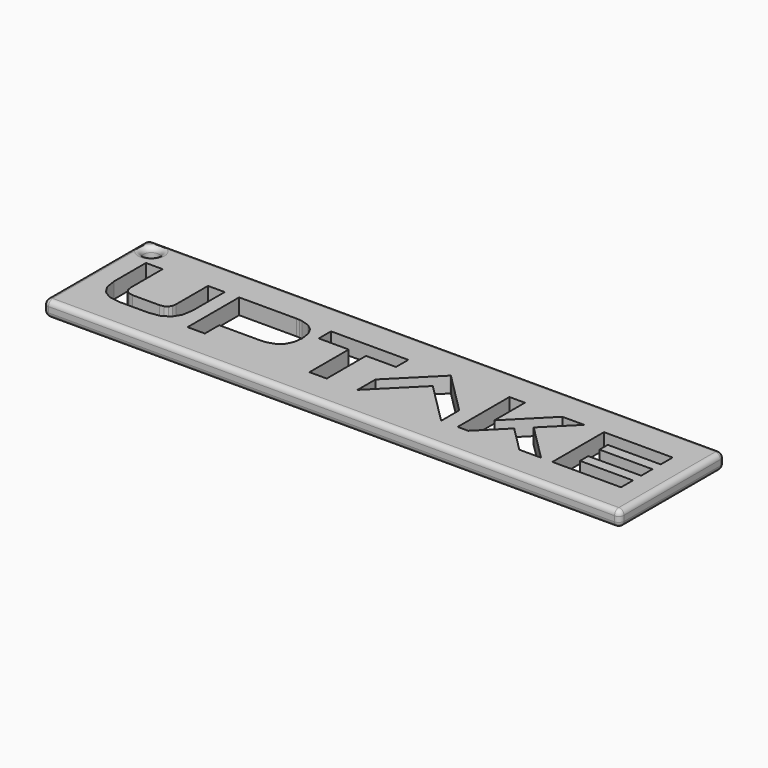
from build123d import *

# Parameters (mm, degrees)
F0_W         = 139.7
F0_H         = 31.75
F1_DEPTH     = 3.81
F3_D         = 3.81
F4_T1_DEPTH  = 137.1580686292
F4_T3_DEPTH  = 29.2080686292
F4_T5_DEPTH  = 1.2680686292
F4_S9_W      = 1.3985022539
F4_S9_H      = 1.3985022539
F4_T10_DEPTH = 1.398502254
F4_S15_W     = 1.398502254
F4_S15_H     = 1.3985022539
F4_T16_DEPTH = 1.398502254
F4_S21_W     = 1.398502254
F4_S21_H     = 1.3985022539
F4_T22_DEPTH = 1.398502254
F4_S27_W     = 1.398502254
F4_S27_H     = 1.3985022539
F4_T28_DEPTH = 1.398502254
F4_S33_W     = 1.398502254
F4_S33_H     = 1.3985022539
F4_T34_DEPTH = 1.398502254
F4_S39_W     = 1.3985022539
F4_S39_H     = 1.3985022539
F4_T40_DEPTH = 1.398502254
F4_S45_W     = 1.398502254
F4_S45_H     = 1.3985022539
F4_T46_DEPTH = 1.398502254
F4_S51_W     = 1.398502254
F4_S51_H     = 1.3985022539
F4_T52_DEPTH = 1.398502254


# Not quite as in the source:
# - a fillet or chamfer that OpenCascade refuses, or shapes differently, is made with other operations: its cross-section is extruded or revolved along the edge and cut away or added


with BuildPart() as f1:
    # F0 (on Top) → F1 (new body)
    with BuildSketch(Plane.XY):
        with Locations((-0.1280346769, -0.0092075206)):
            Rectangle(F0_W, F0_H)
        Polygon((-50.8588471136, -7.8903307544), (-58.0754704074, -7.8903307544), (-60.6254633669, -7.4858431206), (-62.468415754, -6.3530423178), (-63.5997030914, -4.5040080421), (-64.0132995446, -1.9540431098), (-64.0132995446, 7.7319951261), (-59.9625094803, 7.7319951261), (-59.9625094803, -1.9540431098), (-59.8013254183, -2.8937089149), (-59.3801336111, -3.5658276752), (-58.6989340587, -3.9824510591), (-57.7501033799, -4.1649357448), (-51.1842701954, -4.1649357448), (-50.2490887321, -3.985506017), (-49.5542119371, -3.5567188558), (-49.122369818, -2.8785462341), (-48.9718360679, -1.9540431098), (-48.9718360679, 7.7319951261), (-44.9210179765, 7.7319951261), (-44.9210179765, -1.9540431098), (-45.3361278951, -4.5040080421), (-46.4674432595, -6.3530423178), (-48.3103956467, -7.4858431206), align=None, mode=Mode.SUBTRACT)
        Polygon((-26.8019506959, 7.701585683), (-26.0841757304, 7.6164672694), (-24.1589917248, 7.0325499078), (-22.759036257, 5.8936391893), (-21.904208594, 4.23011653), (-21.6135671886, 2.0739608925), (-21.8904752971, -0.0305127052), (-22.7024214413, -1.6559745132), (-24.0314682537, -2.7842629469), (-25.8515504975, -3.3970482592), (-26.6057607405, -3.4928450117), (-27.5516765971, -3.5369316974), (-37.2375746972, -3.5369316974), (-37.2375746972, -7.8903307544), (-41.428304254, -7.8903307544), (-41.428304254, 7.7319951261), (-27.5516765971, 7.7319951261), align=None, mode=Mode.SUBTRACT)
        Polygon((-7.6975333777, -7.8903307544), (-11.888150826, -7.8903307544), (-11.888150826, 4.0066001164), (-19.1536254187, 4.0066001164), (-19.1536254187, 7.7319951261), (-0.432058785, 7.7319951261), (-0.432058785, 4.0066001164), (-7.6975333777, 4.0066001164), align=None, mode=Mode.SUBTRACT)
        Polygon((10.015616885, 7.6012485343), (19.9630081687, -2.3478524046), (20.0179413562, -2.4025894022), (20.0179413562, -2.4801124617), (20.0179413562, -7.4341610809), (20.0179413562, -7.8827073733), (19.7001136284, -7.5649356997), (9.8833288008, 2.251877155), (0.064862345, -7.5649356997), (-0.2512837546, -7.8827073733), (-0.2512837546, -7.4341610809), (-0.2512837546, -2.4801124617), (-0.2512837546, -2.4025894022), (-0.1966308384, -2.3478524046), (9.7510407166, 7.6012485343), (9.8833288008, 7.7319951261), align=None, mode=Mode.SUBTRACT)
        Polygon((35.4017563051, 0.9335367087), (44.2255396868, -7.8903307544), (38.9642856246, -7.8903307544), (32.771129274, -1.6970342682), (26.5776926521, -7.8903307544), (24.0157321054, -7.8903307544), (24.0157321054, 7.8019508587), (27.7649221539, 7.8019508587), (27.7649221539, -1.4415949462), (36.891678881, 7.7319951261), (42.1997382612, 7.7319951261), align=None, mode=Mode.SUBTRACT)
        Polygon((63.6292868227, -4.2804916286), (63.6292868227, -7.8979261084), (46.9822888321, -7.8979261084), (46.9822888321, 7.7319951261), (63.6292868227, 7.7319951261), (63.6292868227, 4.1145886734), (50.7897753245, 4.1145886734), (50.7897753245, 1.6086823996), (63.6292868227, 1.6086823996), (63.6292868227, -1.7973994439), (50.7897753245, -1.7973994439), (50.7897753245, -4.2804916286), align=None, mode=Mode.SUBTRACT)
    extrude(amount=F1_DEPTH)

    # F3 (through all)
    with Locations(Plane.XY.offset(3.81)):
        with Locations((-66.1680346769, 12.0557924794)):
            Hole(F3_D / 2)

    # F4: fillet of radius 1.27 on 14 edges, made by hand

    # F4_s2 → F4_t1 (cut)
    with BuildSketch(Plane.YZ.offset(-68.7070689915)):
        with BuildLine():
            ThreePointArc((15.8661924794, 2.5390343146), (15.4938180915, 3.4380256121), (14.5948267939, 3.8104))
            Line((14.5948267939, 3.8104), (14.5948267939, 3.9375365685))
            ThreePointArc((14.5948267939, 3.9375365685), (15.2303096367, 3.9371365685), (15.8657924794, 3.9371365685))
            Line((15.8657924794, 3.9371365685), (15.9929290479, 3.81))
            ThreePointArc((15.9929290479, 3.81), (15.9929290479, 3.1745171573), (15.9933290479, 2.5390343146))
            Line((15.9933290479, 2.5390343146), (15.8661924794, 2.5390343146))
        make_face()
        with BuildLine():
            ThreePointArc((-14.6132418352, 3.8104), (-15.5122331327, 3.4380256121), (-15.8846075206, 2.5390343146))
            Line((-15.8846075206, 2.5390343146), (-16.0117440892, 2.5390343146))
            ThreePointArc((-16.0117440892, 2.5390343146), (-16.0113440892, 3.1745171573), (-16.0113440892, 3.81))
            Line((-16.0113440892, 3.81), (-15.8842075206, 3.9371365685))
            ThreePointArc((-15.8842075206, 3.9371365685), (-15.2487246779, 3.9371365685), (-14.6132418352, 3.9375365685))
            Line((-14.6132418352, 3.9375365685), (-14.6132418352, 3.8104))
        make_face()
        with BuildLine():
            ThreePointArc((15.8661924794, 1.2709656854), (15.4938180915, 0.3719743879), (14.5948267939, -0.0004))
            Line((14.5948267939, -0.0004), (14.5948267939, -0.1275365685))
            ThreePointArc((14.5948267939, -0.1275365685), (15.2303096367, -0.1271365685), (15.8657924794, -0.1271365685))
            Line((15.8657924794, -0.1271365685), (15.9929290479, 0))
            ThreePointArc((15.9929290479, 0), (15.9929290479, 0.6354828427), (15.9933290479, 1.2709656854))
            Line((15.9933290479, 1.2709656854), (15.8661924794, 1.2709656854))
        make_face()
        with BuildLine():
            ThreePointArc((-14.6132418352, -0.0004), (-15.5122331327, 0.3719743879), (-15.8846075206, 1.2709656854))
            Line((-15.8846075206, 1.2709656854), (-16.0117440892, 1.2709656854))
            ThreePointArc((-16.0117440892, 1.2709656854), (-16.0113440892, 0.6354828427), (-16.0113440892, 0))
            Line((-16.0113440892, 0), (-15.8842075206, -0.1271365685))
            ThreePointArc((-15.8842075206, -0.1271365685), (-15.2487246779, -0.1271365685), (-14.6132418352, -0.1275365685))
            Line((-14.6132418352, -0.1275365685), (-14.6132418352, -0.0004))
        make_face()
    extrude(amount=F4_T1_DEPTH, mode=Mode.SUBTRACT)

    # F4_s4 → F4_t3 (cut)
    with BuildSketch(Plane.XZ.offset(-14.5948267939)):
        with BuildLine():
            ThreePointArc((-69.9784346769, 2.5390343146), (-69.606060289, 3.4380256121), (-68.7070689915, 3.8104))
            Line((-68.7070689915, 3.8104), (-68.7070689915, 3.9375365685))
            ThreePointArc((-68.7070689915, 3.9375365685), (-69.3425518342, 3.9371365685), (-69.9780346769, 3.9371365685))
            Line((-69.9780346769, 3.9371365685), (-70.1051712455, 3.81))
            ThreePointArc((-70.1051712455, 3.81), (-70.1051712455, 3.1745171573), (-70.1055712455, 2.5390343146))
            Line((-70.1055712455, 2.5390343146), (-69.9784346769, 2.5390343146))
        make_face()
        with BuildLine():
            ThreePointArc((69.7223653231, 2.5390343146), (69.3499909352, 3.4380256121), (68.4509996377, 3.8104))
            Line((68.4509996377, 3.8104), (68.4509996377, 3.9375365685))
            ThreePointArc((68.4509996377, 3.9375365685), (69.0864824804, 3.9371365685), (69.7219653231, 3.9371365685))
            Line((69.7219653231, 3.9371365685), (69.8491018916, 3.81))
            ThreePointArc((69.8491018916, 3.81), (69.8491018916, 3.1745171573), (69.8495018916, 2.5390343146))
            Line((69.8495018916, 2.5390343146), (69.7223653231, 2.5390343146))
        make_face()
        with BuildLine():
            ThreePointArc((69.7223653231, 1.2709656854), (69.3499909352, 0.3719743879), (68.4509996377, -0.0004))
            Line((68.4509996377, -0.0004), (68.4509996377, -0.1275365685))
            ThreePointArc((68.4509996377, -0.1275365685), (69.0864824804, -0.1271365685), (69.7219653231, -0.1271365685))
            Line((69.7219653231, -0.1271365685), (69.8491018916, 0))
            ThreePointArc((69.8491018916, 0), (69.8491018916, 0.6354828427), (69.8495018916, 1.2709656854))
            Line((69.8495018916, 1.2709656854), (69.7223653231, 1.2709656854))
        make_face()
        with BuildLine():
            ThreePointArc((-69.9784346769, 1.2709656854), (-69.606060289, 0.3719743879), (-68.7070689915, -0.0004))
            Line((-68.7070689915, -0.0004), (-68.7070689915, -0.1275365685))
            ThreePointArc((-68.7070689915, -0.1275365685), (-69.3425518342, -0.1271365685), (-69.9780346769, -0.1271365685))
            Line((-69.9780346769, -0.1271365685), (-70.1051712455, 0))
            ThreePointArc((-70.1051712455, 0), (-70.1051712455, 0.6354828427), (-70.1055712455, 1.2709656854))
            Line((-70.1055712455, 1.2709656854), (-69.9784346769, 1.2709656854))
        make_face()
    extrude(amount=F4_T3_DEPTH, mode=Mode.SUBTRACT)

    # F4_s6 → F4_t5 (cut)
    with BuildSketch(Plane.XY.offset(1.2709656854)):
        with BuildLine():
            ThreePointArc((-68.7070689915, 15.8661924794), (-69.606060289, 15.4938180915), (-69.9784346769, 14.5948267939))
            Line((-69.9784346769, 14.5948267939), (-70.1055712455, 14.5948267939))
            ThreePointArc((-70.1055712455, 14.5948267939), (-70.1051712455, 15.2303096367), (-70.1051712455, 15.8657924794))
            Line((-70.1051712455, 15.8657924794), (-69.9780346769, 15.9929290479))
            ThreePointArc((-69.9780346769, 15.9929290479), (-69.3425518342, 15.9929290479), (-68.7070689915, 15.9933290479))
            Line((-68.7070689915, 15.9933290479), (-68.7070689915, 15.8661924794))
        make_face()
        with BuildLine():
            ThreePointArc((-69.9784346769, -14.6132418352), (-69.606060289, -15.5122331327), (-68.7070689915, -15.8846075206))
            Line((-68.7070689915, -15.8846075206), (-68.7070689915, -16.0117440892))
            ThreePointArc((-68.7070689915, -16.0117440892), (-69.3425518342, -16.0113440892), (-69.9780346769, -16.0113440892))
            Line((-69.9780346769, -16.0113440892), (-70.1051712455, -15.8842075206))
            ThreePointArc((-70.1051712455, -15.8842075206), (-70.1051712455, -15.2487246779), (-70.1055712455, -14.6132418352))
            Line((-70.1055712455, -14.6132418352), (-69.9784346769, -14.6132418352))
        make_face()
        with BuildLine():
            ThreePointArc((69.7223653231, -14.6132418352), (69.3499909352, -15.5122331327), (68.4509996377, -15.8846075206))
            Line((68.4509996377, -15.8846075206), (68.4509996377, -16.0117440892))
            ThreePointArc((68.4509996377, -16.0117440892), (69.0864824804, -16.0113440892), (69.7219653231, -16.0113440892))
            Line((69.7219653231, -16.0113440892), (69.8491018916, -15.8842075206))
            ThreePointArc((69.8491018916, -15.8842075206), (69.8491018916, -15.2487246779), (69.8495018916, -14.6132418352))
            Line((69.8495018916, -14.6132418352), (69.7223653231, -14.6132418352))
        make_face()
        with BuildLine():
            ThreePointArc((68.4509996377, 15.8661924794), (69.3499909352, 15.4938180915), (69.7223653231, 14.5948267939))
            Line((69.7223653231, 14.5948267939), (69.8495018916, 14.5948267939))
            ThreePointArc((69.8495018916, 14.5948267939), (69.8491018916, 15.2303096367), (69.8491018916, 15.8657924794))
            Line((69.8491018916, 15.8657924794), (69.7219653231, 15.9929290479))
            ThreePointArc((69.7219653231, 15.9929290479), (69.0864824804, 15.9929290479), (68.4509996377, 15.9933290479))
            Line((68.4509996377, 15.9933290479), (68.4509996377, 15.8661924794))
        make_face()
    extrude(amount=F4_T5_DEPTH, mode=Mode.SUBTRACT)


with BuildPart() as f4_tool8:
    # F4_s9 → F4_t10 (new body)
    with BuildSketch(Plane.XZ.offset(-14.5948267939)):
        with Locations((69.1502507646, 3.2382854415)):
            Rectangle(F4_S9_W, F4_S9_H)
    extrude(amount=-F4_T10_DEPTH)

    # F4_s11 → F4_t12 (revolve, cut)
    with BuildSketch(Plane(origin=(68.4509996377, 14.5948267939, 2.5390343146), x_dir=(-0.7071067812, 0, -0.7071067812), z_dir=(0.7071067812, 0, -0.7071067812))):
        with BuildLine():
            ThreePointArc((0, -1.2713656854), (1.2713656854, 0), (0, 1.2713656854))
            Line((0, 1.2713656854), (0, -1.2713656854))
        make_face()
    revolve(axis=Axis((68.4509996377, 14.5948267939, 2.5390343146), (0, 1, 0)), mode=Mode.SUBTRACT)


with BuildPart() as f1_1:
    add(f1.part)

    # F4_t7: cut F4_tool8
    add(f4_tool8.part, mode=Mode.SUBTRACT)


with BuildPart() as f4_tool14:
    # F4_s15 → F4_t16 (new body)
    with BuildSketch(Plane.XZ.offset(-14.5948267939)):
        with Locations((-69.4063201185, 3.2382854415)):
            Rectangle(F4_S15_W, F4_S15_H)
    extrude(amount=-F4_T16_DEPTH)

    # F4_s17 → F4_t18 (revolve, cut)
    with BuildSketch(Plane(origin=(-68.7070689915, 14.5948267939, 2.5390343146), x_dir=(0.7071067812, 0, -0.7071067812), z_dir=(0.7071067812, 0, 0.7071067812))):
        with BuildLine():
            ThreePointArc((0, -1.2713656854), (1.2713656854, 0), (0, 1.2713656854))
            Line((0, 1.2713656854), (0, -1.2713656854))
        make_face()
    revolve(axis=Axis((-68.7070689915, 14.5948267939, 2.5390343146), (0, 1, 0)), mode=Mode.SUBTRACT)


with BuildPart() as f1_2:
    add(f1_1.part)

    # F4_t13: cut F4_tool14
    add(f4_tool14.part, mode=Mode.SUBTRACT)


with BuildPart() as f4_tool20:
    # F4_s21 → F4_t22 (new body)
    with BuildSketch(Plane.YZ.offset(-68.7070689915)):
        with Locations((-15.3124929622, 3.2382854415)):
            Rectangle(F4_S21_W, F4_S21_H)
    extrude(amount=-F4_T22_DEPTH)

    # F4_s23 → F4_t24 (revolve, cut)
    with BuildSketch(Plane(origin=(-68.7070689915, -14.6132418352, 2.5390343146), x_dir=(0, 0.7071067812, -0.7071067812), z_dir=(0, 0.7071067812, 0.7071067812))):
        with BuildLine():
            ThreePointArc((0, -1.2713656854), (1.2713656854, 0), (0, 1.2713656854))
            Line((0, 1.2713656854), (0, -1.2713656854))
        make_face()
    revolve(axis=Axis((-68.7070689915, -14.6132418352, 2.5390343146), (-1, 0, 0)), mode=Mode.SUBTRACT)


with BuildPart() as f1_3:
    add(f1_2.part)

    # F4_t19: cut F4_tool20
    add(f4_tool20.part, mode=Mode.SUBTRACT)


with BuildPart() as f4_tool26:
    # F4_s27 → F4_t28 (new body)
    with BuildSketch(Plane.YZ.offset(68.4509996377)):
        with Locations((-15.3124929622, 3.2382854415)):
            Rectangle(F4_S27_W, F4_S27_H)
    extrude(amount=F4_T28_DEPTH)

    # F4_s29 → F4_t30 (revolve, cut)
    with BuildSketch(Plane(origin=(68.4509996377, -14.6132418352, 2.5390343146), x_dir=(0, 0.7071067812, -0.7071067812), z_dir=(0, -0.7071067812, -0.7071067812))):
        with BuildLine():
            ThreePointArc((0, -1.2713656854), (1.2713656854, 0), (0, 1.2713656854))
            Line((0, 1.2713656854), (0, -1.2713656854))
        make_face()
    revolve(axis=Axis((68.4509996377, -14.6132418352, 2.5390343146), (1, 0, 0)), mode=Mode.SUBTRACT)


with BuildPart() as f1_4:
    add(f1_3.part)

    # F4_t25: cut F4_tool26
    add(f4_tool26.part, mode=Mode.SUBTRACT)


with BuildPart() as f4_tool32:
    # F4_s33 → F4_t34 (new body)
    with BuildSketch(Plane.YZ.offset(68.4509996377)):
        with Locations((-15.3124929622, 0.5717145584)):
            Rectangle(F4_S33_W, F4_S33_H)
    extrude(amount=F4_T34_DEPTH)

    # F4_s35 → F4_t36 (revolve, cut)
    with BuildSketch(Plane(origin=(68.4509996377, -14.6132418352, 1.2709656854), x_dir=(0, 0.7071067812, 0.7071067812), z_dir=(0, 0.7071067812, -0.7071067812))):
        with BuildLine():
            ThreePointArc((0, -1.2713656854), (1.2713656854, 0), (0, 1.2713656854))
            Line((0, 1.2713656854), (0, -1.2713656854))
        make_face()
    revolve(axis=Axis((68.4509996377, -14.6132418352, 1.2709656854), (1, 0, 0)), mode=Mode.SUBTRACT)


with BuildPart() as f1_5:
    add(f1_4.part)

    # F4_t31: cut F4_tool32
    add(f4_tool32.part, mode=Mode.SUBTRACT)


with BuildPart() as f4_tool38:
    # F4_s39 → F4_t40 (new body)
    with BuildSketch(Plane.XZ.offset(-14.5948267939)):
        with Locations((69.1502507646, 0.5717145584)):
            Rectangle(F4_S39_W, F4_S39_H)
    extrude(amount=-F4_T40_DEPTH)

    # F4_s41 → F4_t42 (revolve, cut)
    with BuildSketch(Plane(origin=(68.4509996377, 14.5948267939, 1.2709656854), x_dir=(-0.7071067812, 0, 0.7071067812), z_dir=(-0.7071067812, 0, -0.7071067812))):
        with BuildLine():
            ThreePointArc((0, -1.2713656854), (1.2713656854, 0), (0, 1.2713656854))
            Line((0, 1.2713656854), (0, -1.2713656854))
        make_face()
    revolve(axis=Axis((68.4509996377, 14.5948267939, 1.2709656854), (0, 1, 0)), mode=Mode.SUBTRACT)


with BuildPart() as f1_6:
    add(f1_5.part)

    # F4_t37: cut F4_tool38
    add(f4_tool38.part, mode=Mode.SUBTRACT)


with BuildPart() as f4_tool44:
    # F4_s45 → F4_t46 (new body)
    with BuildSketch(Plane.XZ.offset(-14.5948267939)):
        with Locations((-69.4063201185, 0.5717145584)):
            Rectangle(F4_S45_W, F4_S45_H)
    extrude(amount=-F4_T46_DEPTH)

    # F4_s47 → F4_t48 (revolve, cut)
    with BuildSketch(Plane(origin=(-68.7070689915, 14.5948267939, 1.2709656854), x_dir=(0.7071067812, 0, 0.7071067812), z_dir=(-0.7071067812, 0, 0.7071067812))):
        with BuildLine():
            ThreePointArc((0, -1.2713656854), (1.2713656854, 0), (0, 1.2713656854))
            Line((0, 1.2713656854), (0, -1.2713656854))
        make_face()
    revolve(axis=Axis((-68.7070689915, 14.5948267939, 1.2709656854), (0, 1, 0)), mode=Mode.SUBTRACT)


with BuildPart() as f1_7:
    add(f1_6.part)

    # F4_t43: cut F4_tool44
    add(f4_tool44.part, mode=Mode.SUBTRACT)


with BuildPart() as f4_tool50:
    # F4_s51 → F4_t52 (new body)
    with BuildSketch(Plane.YZ.offset(-68.7070689915)):
        with Locations((-15.3124929622, 0.5717145584)):
            Rectangle(F4_S51_W, F4_S51_H)
    extrude(amount=-F4_T52_DEPTH)

    # F4_s53 → F4_t54 (revolve, cut)
    with BuildSketch(Plane(origin=(-68.7070689915, -14.6132418352, 1.2709656854), x_dir=(0, 0.7071067812, 0.7071067812), z_dir=(0, -0.7071067812, 0.7071067812))):
        with BuildLine():
            ThreePointArc((0, -1.2713656854), (1.2713656854, 0), (0, 1.2713656854))
            Line((0, 1.2713656854), (0, -1.2713656854))
        make_face()
    revolve(axis=Axis((-68.7070689915, -14.6132418352, 1.2709656854), (-1, 0, 0)), mode=Mode.SUBTRACT)


with BuildPart() as f1_8:
    add(f1_7.part)

    # F4_t49: cut F4_tool50
    add(f4_tool50.part, mode=Mode.SUBTRACT)

    # F4_s55 → F4_t56 (revolve, cut)
    with BuildSketch(Plane.XZ.offset(-12.0557924794)):
        with BuildLine():
            ThreePointArc((-62.9920689915, -0.0004), (-63.891060289, 0.3719743879), (-64.2634346769, 1.2709656854))
            Line((-64.2634346769, 1.2709656854), (-64.3905712455, 1.2709656854))
            ThreePointArc((-64.3905712455, 1.2709656854), (-64.3901712455, 0.6354828427), (-64.3901712455, 0))
            Line((-64.3901712455, 0), (-64.2630346769, -0.1271365685))
            ThreePointArc((-64.2630346769, -0.1271365685), (-63.6275518342, -0.1271365685), (-62.9920689915, -0.1275365685))
            Line((-62.9920689915, -0.1275365685), (-62.9920689915, -0.0004))
        make_face()
    revolve(axis=Axis((-66.1680346769, 12.0557924794, 0), (0, 0, 1)), mode=Mode.SUBTRACT)

    # F4_s57 → F4_t58 (revolve, cut)
    with BuildSketch(Plane.XZ.offset(-12.0557924794)):
        with BuildLine():
            ThreePointArc((-62.9920689915, 3.8104), (-63.891060289, 3.4380256121), (-64.2634346769, 2.5390343146))
            Line((-64.2634346769, 2.5390343146), (-64.3905712455, 2.5390343146))
            ThreePointArc((-64.3905712455, 2.5390343146), (-64.3901712455, 3.1745171573), (-64.3901712455, 3.81))
            Line((-64.3901712455, 3.81), (-64.2630346769, 3.9371365685))
            ThreePointArc((-64.2630346769, 3.9371365685), (-63.6275518342, 3.9371365685), (-62.9920689915, 3.9375365685))
            Line((-62.9920689915, 3.9375365685), (-62.9920689915, 3.8104))
        make_face()
    revolve(axis=Axis((-66.1680346769, 12.0557924794, 3.81), (0, 0, 1)), mode=Mode.SUBTRACT)


solid = f1_8.part
